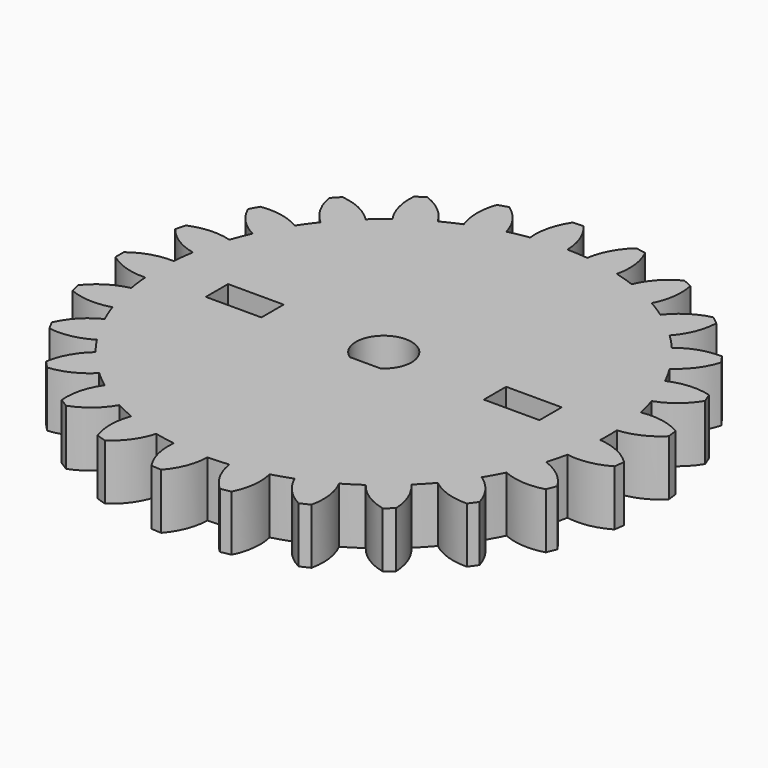
from build123d import *

# Parameters (mm, degrees)
F1_W     = 6
F1_H     = 3
F2_DEPTH = 6


# Not quite as in the source:
# - a feature names something its author has since deleted; it is built from what else it names


with BuildPart() as f2:
    # F1 (on Top) → F2 (new body)
    with BuildSketch(Plane.XY):
        with BuildLine():
            ThreePointArc((2.6492001042, 24.1328040773), (1.5244142797, 24.2298711291), (0.3963319999, 24.2745425245))
            ThreePointArc((0.3963319999, 24.2745425245), (-0.0481990645, 26.5171542751), (-1.2314510555, 28.4733828039))
            Line((-1.2314510555, 28.4733828039), (-2.3469204412, 28.4032034187))
            ThreePointArc((-2.3469204412, 28.4032034187), (-3.2756616898, 26.314099538), (-3.4356137115, 24.0334569351))
            ThreePointArc((-3.4356137115, 24.0334569351), (-4.5492019152, 23.8477515871), (-5.6529527401, 23.6104768936))
            ThreePointArc((-5.6529527401, 23.6104768936), (-6.6412329068, 25.672082492), (-8.2738051128, 27.2725897002))
            Line((-8.2738051128, 27.2725897002), (-9.3367770732, 26.9272091737))
            ThreePointArc((-9.3367770732, 26.9272091737), (-9.7168011992, 24.6727697767), (-9.3045552825, 22.4239993048))
            ThreePointArc((-9.3045552825, 22.4239993048), (-10.336975023, 21.9671901071), (-11.3470416693, 21.4628781663))
            ThreePointArc((-11.3470416693, 21.4628781663), (-12.8169736609, 23.2139393506), (-14.796285566, 24.358159484))
            Line((-14.796285566, 24.358159484), (-15.7399696634, 23.7592793451))
            ThreePointArc((-15.7399696634, 23.7592793451), (-15.5473983534, 21.4811591503), (-14.5888574253, 19.4055593285))
            ThreePointArc((-14.5888574253, 19.4055593285), (-15.4752379733, 18.7063492829), (-16.3281542389, 17.9666878688))
            ThreePointArc((-16.3281542389, 17.9666878688), (-18.1873768224, 19.297179025), (-20.3890609801, 19.9132165245))
            Line((-20.3890609801, 19.9132165245), (-21.1541620721, 19.0984666146))
            ThreePointArc((-21.1541620721, 19.0984666146), (-20.4010952897, 16.9398082923), (-18.9564880021, 15.1677966909))
            ThreePointArc((-18.9564880021, 15.1677966909), (-19.6411348079, 14.2701197362), (-20.283308827, 13.3415844957))
            ThreePointArc((-20.283308827, 13.3415844957), (-22.4150002096, 14.1679059711), (-24.7007167071, 14.217052935))
            Line((-24.7007167071, 14.217052935), (-25.2391606782, 13.2376269875))
            ThreePointArc((-25.2391606782, 13.2376269875), (-23.972916379, 11.334066979), (-22.1330127205, 9.9769856039))
            ThreePointArc((-22.1330127205, 9.9769856039), (-22.5729069074, 8.9372460846), (-22.9639885246, 7.8781803018))
            ThreePointArc((-22.9639885246, 7.8781803018), (-25.234206697, 8.1484112791), (-27.4603355605, 7.6275796229))
            Line((-27.4603355605, 7.6275796229), (-27.7382899958, 6.5450185722))
            ThreePointArc((-27.7382899958, 6.5450185722), (-26.038430966, 5.0161645537), (-23.9188388502, 4.1592838187))
            ThreePointArc((-23.9188388502, 4.1592838187), (-24.0863402486, 3.0428123926), (-24.2017563676, 1.9197610656))
            ThreePointArc((-24.2017563676, 1.9197610656), (-26.4678551727, 1.6169219388), (-28.4945205386, 0.5588374309))
            Line((-28.4945205386, 0.5588374309), (-28.4945205386, -0.5588374309))
            ThreePointArc((-28.4945205386, -0.5588374309), (-26.4678551727, -1.6169219388), (-24.2017563676, -1.9197610656))
            ThreePointArc((-24.2017563676, -1.9197610656), (-24.0863402486, -3.0428123926), (-23.9188388502, -4.1592838187))
            ThreePointArc((-23.9188388502, -4.1592838187), (-26.038430966, -5.0161645537), (-27.7382899958, -6.5450185722))
            Line((-27.7382899958, -6.5450185722), (-27.4603355605, -7.6275796229))
            ThreePointArc((-27.4603355605, -7.6275796229), (-25.234206697, -8.1484112791), (-22.9639885246, -7.8781803018))
            ThreePointArc((-22.9639885246, -7.8781803018), (-22.5729069074, -8.9372460846), (-22.1330127205, -9.9769856039))
            ThreePointArc((-22.1330127205, -9.9769856039), (-23.972916379, -11.334066979), (-25.2391606782, -13.2376269875))
            Line((-25.2391606782, -13.2376269875), (-24.7007167071, -14.217052935))
            ThreePointArc((-24.7007167071, -14.217052935), (-22.4150002096, -14.1679059711), (-20.283308827, -13.3415844957))
            ThreePointArc((-20.283308827, -13.3415844957), (-19.6411348079, -14.2701197362), (-18.9564880021, -15.1677966909))
            ThreePointArc((-18.9564880021, -15.1677966909), (-20.4010952897, -16.9398082923), (-21.1541620721, -19.0984666146))
            Line((-21.1541620721, -19.0984666146), (-20.3890609801, -19.9132165245))
            ThreePointArc((-20.3890609801, -19.9132165245), (-18.1873768224, -19.297179025), (-16.3281542389, -17.9666878688))
            ThreePointArc((-16.3281542389, -17.9666878688), (-15.4752379733, -18.7063492829), (-14.5888574253, -19.4055593285))
            ThreePointArc((-14.5888574253, -19.4055593285), (-15.5473983534, -21.4811591503), (-15.7399696634, -23.7592793451))
            Line((-15.7399696634, -23.7592793451), (-14.796285566, -24.358159484))
            ThreePointArc((-14.796285566, -24.358159484), (-12.8169736609, -23.2139393506), (-11.3470416693, -21.4628781663))
            ThreePointArc((-11.3470416693, -21.4628781663), (-10.336975023, -21.9671901071), (-9.3045552825, -22.4239993048))
            ThreePointArc((-9.3045552825, -22.4239993048), (-9.7168011992, -24.6727697767), (-9.3367770732, -26.9272091737))
            Line((-9.3367770732, -26.9272091737), (-8.2738051128, -27.2725897002))
            ThreePointArc((-8.2738051128, -27.2725897002), (-6.6412329068, -25.672082492), (-5.6529527401, -23.6104768936))
            ThreePointArc((-5.6529527401, -23.6104768936), (-4.5492019152, -23.8477515871), (-3.4356137115, -24.0334569351))
            ThreePointArc((-3.4356137115, -24.0334569351), (-3.2756616898, -26.314099538), (-2.3469204412, -28.4032034187))
            Line((-2.3469204412, -28.4032034187), (-1.2314510555, -28.4733828039))
            ThreePointArc((-1.2314510555, -28.4733828039), (-0.0481990645, -26.5171542751), (0.3963319999, -24.2745425245))
            ThreePointArc((0.3963319999, -24.2745425245), (1.5244142797, -24.2298711291), (2.6492001042, -24.1328040773))
            ThreePointArc((2.6492001042, -24.1328040773), (3.3712996907, -26.3020176488), (4.7904018334, -28.0945199331))
            Line((4.7904018334, -28.0945199331), (5.8882796006, -27.8850885483))
            ThreePointArc((5.8882796006, -27.8850885483), (6.5478633024, -25.6960557318), (6.4207137427, -23.413349373))
            ThreePointArc((6.4207137427, -23.413349373), (7.502245919, -23.0895387567), (8.5675549344, -22.7157983851))
            ThreePointArc((8.5675549344, -22.7157983851), (9.8064299128, -24.6372832586), (11.626725543, -26.0205544358))
            Line((11.626725543, -26.0205544358), (12.6380279938, -25.544671625))
            ThreePointArc((12.6380279938, -25.544671625), (12.7324993366, -23.2603795034), (12.0416584273, -21.0810093721))
            ThreePointArc((12.0416584273, -21.0810093721), (13.0086838559, -20.4984057469), (13.9475787787, -19.8714755375))
            ThreePointArc((13.9475787787, -19.8714755375), (15.6253860779, -21.4244977518), (17.7324993267, -22.3116218064))
            Line((17.7324993267, -22.3116218064), (18.5936826087, -21.5991890368))
            ThreePointArc((18.5936826087, -21.5991890368), (18.1171056106, -19.3631680851), (16.9059814268, -17.4240720219))
            ThreePointArc((16.9059814268, -17.4240720219), (17.6977383435, -16.6192825162), (18.4512249528, -15.7785547997))
            ThreePointArc((18.4512249528, -15.7785547997), (20.4625417697, -16.8655322574), (22.724074962, -17.2007679224))
            Line((22.724074962, -17.2007679224), (23.3810277626, -16.2965499651))
            ThreePointArc((23.3810277626, -16.2965499651), (22.3633475091, -14.2492976033), (20.7080394374, -12.6723161452))
            ThreePointArc((20.7080394374, -12.6723161452), (21.2747788433, -11.6959086435), (21.7955128043, -10.6942094344))
            ThreePointArc((21.7955128043, -10.6942094344), (24.0139607061, -11.2468433441), (26.2878133942, -11.0091265299))
            Line((26.2878133942, -11.0091265299), (26.6992569527, -9.9699387246))
            ThreePointArc((26.6992569527, -9.9699387246), (25.2044180369, -8.2400913478), (23.2089351714, -7.1243120397))
            ThreePointArc((23.2089351714, -7.1243120397), (23.5150467452, -6.0376378162), (23.7703084279, -4.9379075597))
            ThreePointArc((23.7703084279, -4.9379075597), (26.0564941741, -4.9214739006), (28.199791831, -4.1257412288))
            Line((28.199791831, -4.1257412288), (28.3398736355, -3.0168795672))
            ThreePointArc((28.3398736355, -3.0168795672), (26.4618022841, -1.713129848), (24.251528152, -1.1286612073))
            ThreePointArc((24.251528152, -1.1286612073), (24.2777777778, 0), (24.251528152, 1.1286612073))
            ThreePointArc((24.251528152, 1.1286612073), (26.4618022841, 1.713129848), (28.3398736355, 3.0168795672))
            Line((28.3398736355, 3.0168795672), (28.199791831, 4.1257412288))
            ThreePointArc((28.199791831, 4.1257412288), (26.0564941741, 4.9214739006), (23.7703084279, 4.9379075597))
            ThreePointArc((23.7703084279, 4.9379075597), (23.5150467452, 6.0376378162), (23.2089351714, 7.1243120397))
            ThreePointArc((23.2089351714, 7.1243120397), (25.2044180369, 8.2400913478), (26.6992569527, 9.9699387246))
            Line((26.6992569527, 9.9699387246), (26.2878133942, 11.0091265299))
            ThreePointArc((26.2878133942, 11.0091265299), (24.0139607061, 11.2468433441), (21.7955128043, 10.6942094344))
            ThreePointArc((21.7955128043, 10.6942094344), (21.2747788433, 11.6959086435), (20.7080394374, 12.6723161452))
            ThreePointArc((20.7080394374, 12.6723161452), (22.3633475091, 14.2492976033), (23.3810277626, 16.2965499651))
            Line((23.3810277626, 16.2965499651), (22.724074962, 17.2007679224))
            ThreePointArc((22.724074962, 17.2007679224), (20.4625417697, 16.8655322574), (18.4512249528, 15.7785547997))
            ThreePointArc((18.4512249528, 15.7785547997), (17.6977383435, 16.6192825162), (16.9059814268, 17.4240720219))
            ThreePointArc((16.9059814268, 17.4240720219), (18.1171056106, 19.3631680851), (18.5936826087, 21.5991890368))
            Line((18.5936826087, 21.5991890368), (17.7324993267, 22.3116218064))
            ThreePointArc((17.7324993267, 22.3116218064), (15.6253860779, 21.4244977518), (13.9475787787, 19.8714755375))
            ThreePointArc((13.9475787787, 19.8714755375), (13.0086838559, 20.4984057469), (12.0416584273, 21.0810093721))
            ThreePointArc((12.0416584273, 21.0810093721), (12.7324993366, 23.2603795034), (12.6380279938, 25.544671625))
            Line((12.6380279938, 25.544671625), (11.626725543, 26.0205544358))
            ThreePointArc((11.626725543, 26.0205544358), (9.8064299128, 24.6372832586), (8.5675549344, 22.7157983851))
            ThreePointArc((8.5675549344, 22.7157983851), (7.502245919, 23.0895387567), (6.4207137427, 23.413349373))
            ThreePointArc((6.4207137427, 23.413349373), (6.5478633024, 25.6960557318), (5.8882796006, 27.8850885483))
            Line((5.8882796006, 27.8850885483), (4.7904018334, 28.0945199331))
            ThreePointArc((4.7904018334, 28.0945199331), (3.3712996907, 26.3020176488), (2.6492001042, 24.1328040773))
        make_face()
        with Locations((-15, 0)):
            Rectangle(F1_W, F1_H, mode=Mode.SUBTRACT)
        with BuildLine():
            Line((1.6583123952, -2.5), (-1.6583123952, -2.5))
            ThreePointArc((-1.6583123952, -2.5), (0, 3), (1.6583123952, -2.5))
        make_face(mode=Mode.SUBTRACT)
        with Locations((15, 0)):
            Rectangle(F1_W, F1_H, mode=Mode.SUBTRACT)
    extrude(amount=F2_DEPTH)


solid = f2.part
